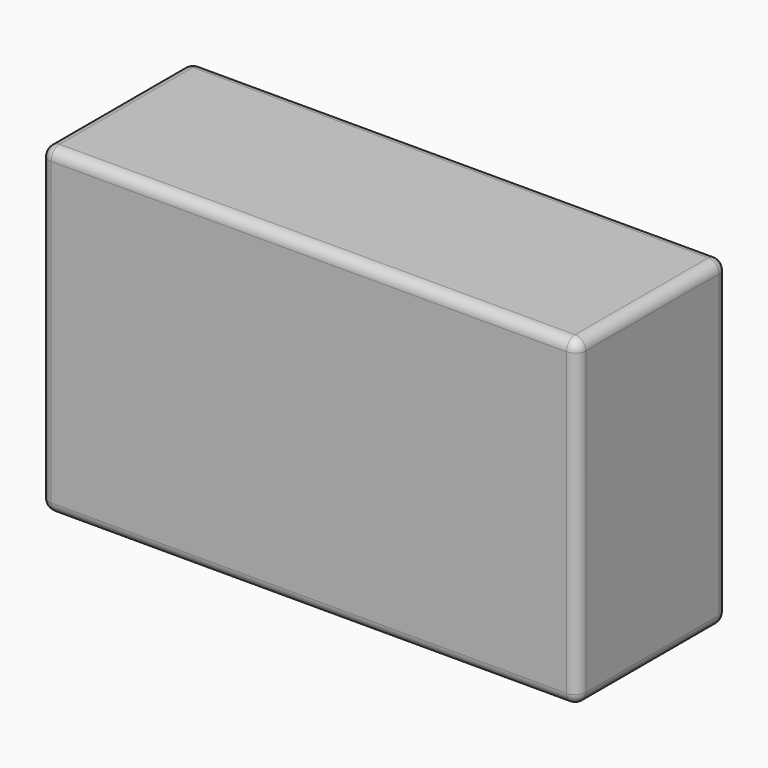
from build123d import *

# Parameters (mm, degrees)
F0_W     = 254
F0_H     = 152.4
F1_DEPTH = 88.9
F2_R     = 5.08
F3_R     = 5.08
F4_R     = 5.08
F5_T     = -2.54


# Not quite as in the source:
# - a shell that OpenCascade refuses in one call is made with other operations: the cavity is built on its own and cut out


with BuildPart() as f1:
    # F0 (on Front) → F1 (new body)
    with BuildSketch(Plane.XZ):
        with Locations((-5.4093236282, -1.1136829853)):
            Rectangle(F0_W, F0_H)
    extrude(amount=F1_DEPTH)

    # F2
    f2_edges = [f1.edges().sort_by_distance(p)[0] for p in [
        (121.590676, -88.9, -1.113683),
        (121.590676, 0, -1.113683),
    ]]
    fillet(f2_edges, radius=F2_R)

    # F3
    f3_edges = [f1.edges().sort_by_distance(p)[0] for p in [
        (-7.949324, -88.9, 75.086317),
        (-7.949324, -88.9, -77.313683),
    ]]
    fillet(f3_edges, radius=F3_R)

    # F4
    f4_edges = [f1.edges().sort_by_distance(p)[0] for p in [
        (-132.409324, 0, -1.113683),
        (-132.409324, -88.9, -1.113683),
    ]]
    fillet(f4_edges, radius=F4_R)

    # F5: a shell. OpenCascade refuses it in one call, so the cavity is built on its own and cut out:
    # the body offset inwards by the wall thickness, plus a prism from it out through each open face.
    f5_core = offset(f1.part, amount=F5_T, mode=Mode.PRIVATE)
    f5_exits = [f5_core.faces().sort_by_distance(p)[0] for p in [
        (-5.409324, -44.45, -74.773683),
    ]]
    add(f5_core, mode=Mode.SUBTRACT)
    extrude(f5_exits, amount=-F5_T, mode=Mode.SUBTRACT)


solid = f1.part
